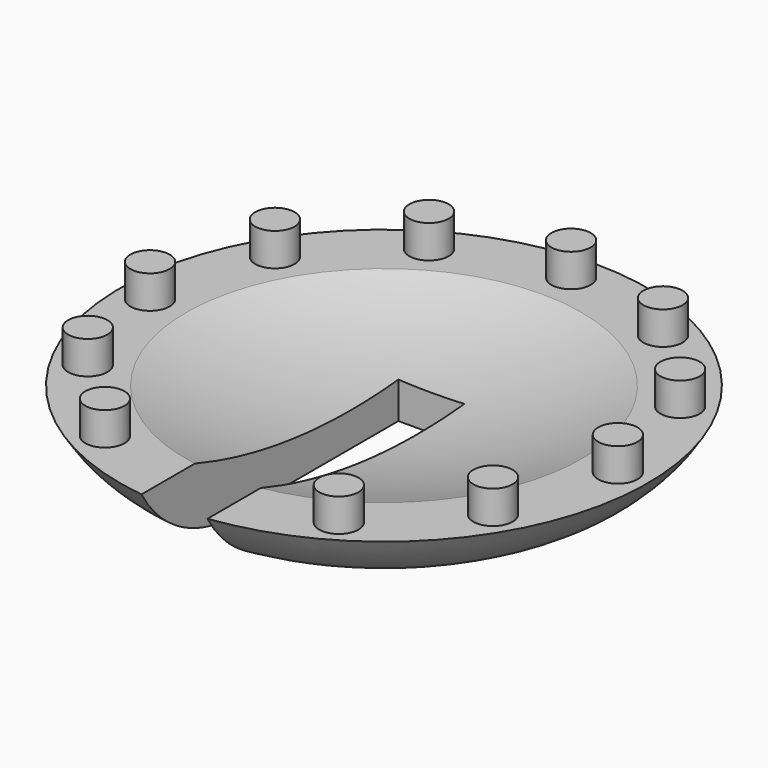
from build123d import *

# Parameters (mm, degrees)
F0_R      = 50.8
F1_DEPTH  = 12.7
F3_R      = 38.1
F4_DEPTH  = 6.35
F6_W      = 12.7
F6_H      = 83.8771756418
F7_DEPTH  = 25.4
F9_R      = 3.81
F10_DEPTH = 41.656
F11_R     = 3.7810776449
F12_DEPTH = 6.35


# Not quite as in the source:
# - a fillet or chamfer that OpenCascade refuses, or shapes differently, is made with other operations: its cross-section is extruded or revolved along the edge and cut away or added


with BuildPart() as f1:
    # F0 (on Top) → F1 (new body)
    with BuildSketch(Plane.XY):
        Circle(F0_R)
    extrude(amount=F1_DEPTH)

    # F2: fillet of radius 25.4 on 1 edges, made by hand

    # F2_s1 → F2_t2 (revolve, cut)
    with BuildSketch(Plane.XZ):
        with BuildLine():
            ThreePointArc((50.8, 12.7), (41.5029547439, 3.4029547439), (28.8029547439, 0))
            Line((28.8029547439, 0), (28.8029547439, -0.508))
            Line((28.8029547439, -0.508), (50.8, -0.508))
            Line((50.8, -0.508), (51.308, 0))
            ThreePointArc((51.308, 0), (51.308, 6.35), (51.2399409051, 12.446))
            Line((51.2399409051, 12.446), (50.8, 12.7))
        make_face()
    revolve(axis=Axis((0, 0, 0), (0, 0, 1)), mode=Mode.SUBTRACT)

    # F3 (on face) → F4 (cut)
    with BuildSketch(Plane.XY.offset(12.7)):
        Circle(F3_R)
    extrude(amount=-F4_DEPTH, mode=Mode.SUBTRACT)

    # F5: fillet of radius 114.3 on 1 edges, made by hand

    # F5_s1 → F5_t2 (revolve)
    with BuildSketch(Plane.XZ):
        with BuildLine():
            ThreePointArc((38.1, 12.7), (19.5828933773, 7.948680132), (0.5328933773, 6.35))
            Line((0.5328933773, 6.35), (38.1, 6.35))
            Line((38.1, 6.35), (38.1, 12.7))
        make_face()
    revolve(axis=Axis((0, 0, 6.35), (0, 0, 1)))

    # F6 (on face) → F7 (cut)
    with BuildSketch(Plane.XY.offset(12.7)):
        with Locations((0, -30.5251618847)):
            Rectangle(F6_W, F6_H)
    extrude(amount=-F7_DEPTH, mode=Mode.SUBTRACT)

    # F9 (on offset) → F10 (cut)
    with BuildSketch(Plane.XZ.offset(-73.406)):
        with Locations((0, 6.35)):
            Circle(F9_R)
    extrude(amount=F10_DEPTH, mode=Mode.SUBTRACT)

    # F11 (on face) → F12 (join)
    with BuildSketch(Plane.XY.offset(12.7)):
        with Locations((-45.025870204, 0)):
            Circle(F11_R)
        with Locations((-38.9935474241, -22.512935102)):
            Circle(F11_R)
        with Locations((-22.512935102, -38.9935474241)):
            Circle(F11_R)
        with Locations((22.512935102, -38.9935474241)):
            Circle(F11_R)
        with Locations((38.9935474241, -22.512935102)):
            Circle(F11_R)
        with Locations((45.025870204, 0)):
            Circle(F11_R)
        with Locations((38.9935474241, 22.512935102)):
            Circle(F11_R)
        with Locations((22.512935102, 38.9935474241)):
            Circle(F11_R)
        with Locations((0, 45.025870204)):
            Circle(F11_R)
        with Locations((-22.512935102, 38.9935474241)):
            Circle(F11_R)
        with Locations((-38.9935474241, 22.512935102)):
            Circle(F11_R)
    extrude(amount=F12_DEPTH)


solid = f1.part
